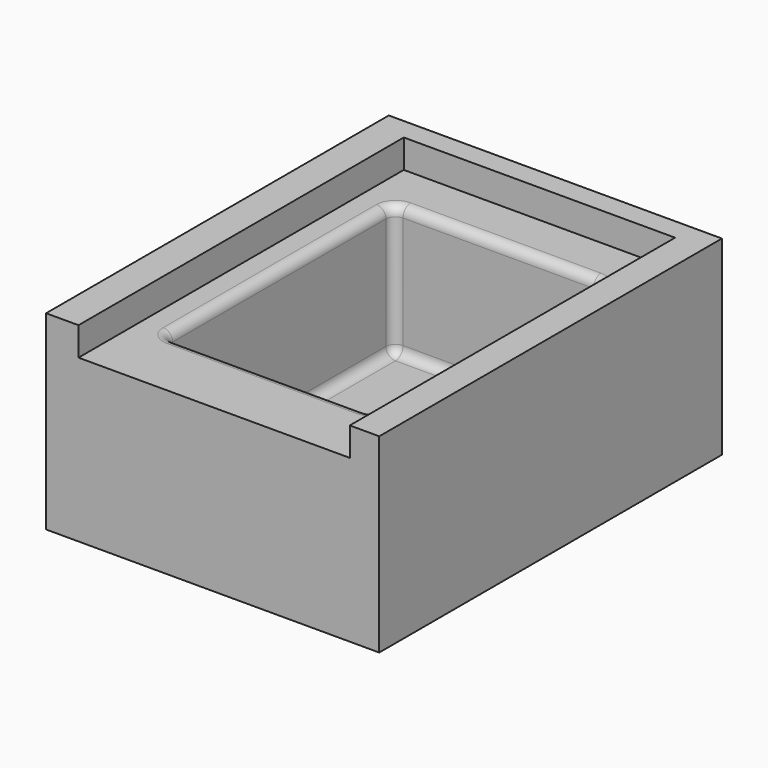
from build123d import *

# Parameters (mm, degrees)
F1_DEPTH = 20
F3_DEPTH = 3
F4_W     = 22
F4_H     = 30
F5_DEPTH = 13.8
F6_W     = 28.5
F6_H     = 2.2146213427
F7_DEPTH = 3
F8_R     = 1


with BuildPart() as f1:
    # F0 (on Top) → F1 (new body)
    with BuildSketch(Plane.XY):
        Polygon((0, 22.5), (-17.5, 22.5), (-17.5, 0), (-14.605, 0), (0, 0), (0, 20.066), align=None)
        Polygon((17.5, 22.5), (0, 22.5), (0, 20.066), (0, 0), (-14.605, 0), (-17.5, 0), (-17.5, -22.5), (17.5, -22.5), align=None)
    extrude(amount=F1_DEPTH)

    # F2 (on face) → F3 (cut)
    with BuildSketch(Plane.XY.offset(20)):
        Polygon((0.1571281302, 20.2146213427), (-14.0928718698, 20.2146213427), (-14.0928718698, 0), (-14.0928718698, -20.2853786573), (14.4071281302, -20.2853786573), (14.4071281302, 20.2146213427), align=None)
    extrude(amount=-F3_DEPTH, mode=Mode.SUBTRACT)

    # F4 (on face) → F5 (cut)
    with BuildSketch(Plane.XY.offset(17)):
        Rectangle(F4_W, F4_H)
    extrude(amount=-F5_DEPTH, mode=Mode.SUBTRACT)

    # F6 (on face) → F7 (cut, through all)
    with BuildSketch(Plane.XY.offset(20)):
        with Locations((0.1571281302, -21.3926893286)):
            Rectangle(F6_W, F6_H)
    extrude(amount=-F7_DEPTH, mode=Mode.SUBTRACT)

    # F8
    f8_edges = [f1.edges().sort_by_distance(p)[0] for p in [
        (-11, 0, 3.2),
        (0, -15, 3.2),
        (0, 15, 3.2),
        (11, 0, 3.2),
        (0, 15, 17),
        (11, 0, 17),
        (-11, 0, 17),
        (0, -15, 17),
        (11, 15, 10.1),
        (-11, 15, 10.1),
        (11, -15, 10.1),
        (-11, -15, 10.1),
    ]]
    fillet(f8_edges, radius=F8_R)


solid = f1.part
